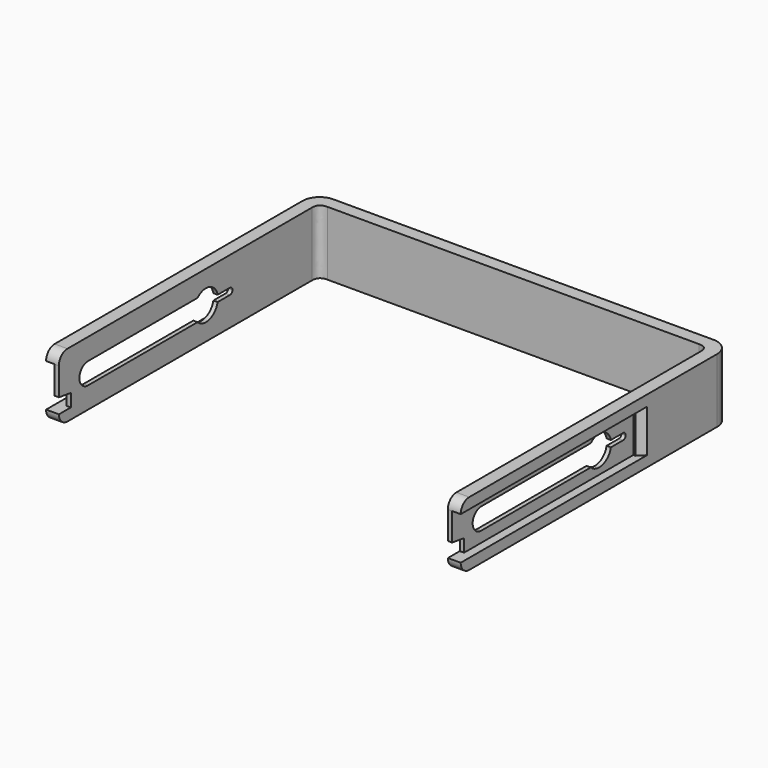
from build123d import *

# Parameters (mm, degrees)
F3_DEPTH      = 15
F4_R          = 2.5
F5_DEPTH      = 48.501
F5_DEPTH_BACK = 48.501
F6_START      = 46.5
F6_DEPTH      = 8.5
F7_START      = 2.5
F7_DEPTH      = 10
F2_W          = 73.5
F2_H          = 1
F8_DEPTH      = 0.6
F9_DEPTH      = 0.8
F10_DEPTH     = 1
F11_R         = 4
F12_T1_DEPTH  = 15


# Not quite as in the source:
# - a fillet or chamfer that OpenCascade refuses, or shapes differently, is made with other operations: its cross-section is extruded or revolved along the edge and cut away or added
# - a pattern or mirror of a feature is missing from the dataset's text; its kind, count and spacing are read off the source's solid


with BuildPart() as f3:
    # F0 (on Top) → F3 (new body)
    with BuildSketch(Plane.XY):
        Polygon((48.5, 0), (-48.5, 0), (-48.5, -79), (-45.5, -79), (-45.5, -3), (45.5, -3), (45.5, -79), (48.5, -79), (48.5, -26), (47, -26), (48.5, -24.5), align=None)
        Polygon((48.5, -26), (48.5, -24.5), (47, -26), align=None)
    extrude(amount=F3_DEPTH)

    # F4
    f4_edges = [f3.edges().sort_by_distance(p)[0] for p in [
        (-47, -79, 15),
        (-47, -79, 0),
        (47, -79, 0),
        (47, -79, 15),
    ]]
    fillet(f4_edges, radius=F4_R)

    # F1 (on Right) → F5 (cut, two sides)
    with BuildSketch(Plane.YZ) as f5_sk:
        with BuildLine():
            ThreePointArc((-38.4494897428, 5), (-39.5, 7.5), (-38.4494897428, 10))
            Line((-38.4494897428, 10), (-70.5, 10))
            ThreePointArc((-70.5, 10), (-68.732233047, 9.267766953), (-68, 7.5))
            ThreePointArc((-68, 7.5), (-68.732233047, 5.732233047), (-70.5, 5))
            Line((-70.5, 5), (-38.4494897428, 5))
        make_face()
        with BuildLine():
            ThreePointArc((-68, 7.5), (-68.732233047, 9.267766953), (-70.5, 10))
            ThreePointArc((-70.5, 10), (-73, 7.5), (-70.5, 5))
            ThreePointArc((-70.5, 5), (-68.732233047, 5.732233047), (-68, 7.5))
        make_face()
        with BuildLine():
            ThreePointArc((-32.5813014172, 6.75), (-32.5203847167, 7.1228031282), (-32.5, 7.5))
            ThreePointArc((-32.5, 7.5), (-32.5203847167, 7.8771968718), (-32.5813014172, 8.25))
            ThreePointArc((-32.5813014172, 8.25), (-34.9997668052, 10.8540324322), (-38.4494897428, 10))
            ThreePointArc((-38.4494897428, 10), (-39.5, 7.5), (-38.4494897428, 5))
            ThreePointArc((-38.4494897428, 5), (-34.9997668052, 4.1459675678), (-32.5813014172, 6.75))
        make_face()
        Polygon((-79, 6), (-79, 2.5), (-75.5, 2.5), (-75.5, 5.5), align=None)
        with BuildLine():
            ThreePointArc((-32.5813014172, 8.25), (-32.5203847167, 7.8771968718), (-32.5, 7.5))
            ThreePointArc((-32.5, 7.5), (-32.5203847167, 7.1228031282), (-32.5813014172, 6.75))
            Line((-32.5813014172, 6.75), (-29, 6.75))
            ThreePointArc((-29, 6.75), (-29.75, 7.5), (-29, 8.25))
            Line((-29, 8.25), (-32.5813014172, 8.25))
        make_face()
        with BuildLine():
            ThreePointArc((-28.25, 7.5), (-28.4696699141, 8.0303300859), (-29, 8.25))
            ThreePointArc((-29, 8.25), (-29.75, 7.5), (-29, 6.75))
            ThreePointArc((-29, 6.75), (-28.4696699141, 6.9696699141), (-28.25, 7.5))
        make_face()
    extrude(amount=-F5_DEPTH, mode=Mode.SUBTRACT)
    extrude(f5_sk.sketch, amount=F5_DEPTH_BACK, mode=Mode.SUBTRACT)

    # F1 (on Right) → F6 (cut)
    with BuildSketch(Plane.YZ.offset(F6_START)):
        Polygon((-79, 6), (-79, 2.5), (-75.5, 2.5), (-75.5, 5.5), align=None)
        Polygon((-75.5, 5.5), (-75.5, 2.5), (-26, 2.5), (-26, 12.5), (-79, 12.5), (-79, 7.5), (-79, 6), align=None)
        with BuildLine():
            ThreePointArc((-38.4494897428, 10), (-34.9997668052, 10.8540324322), (-32.5813014172, 8.25))
            Line((-32.5813014172, 8.25), (-29, 8.25))
            ThreePointArc((-29, 8.25), (-28.4696699141, 8.0303300859), (-28.25, 7.5))
            ThreePointArc((-28.25, 7.5), (-28.4696699141, 6.9696699141), (-29, 6.75))
            Line((-29, 6.75), (-32.5813014172, 6.75))
            ThreePointArc((-32.5813014172, 6.75), (-34.9997668052, 4.1459675678), (-38.4494897428, 5))
            Line((-38.4494897428, 5), (-70.5, 5))
            ThreePointArc((-70.5, 5), (-73, 7.5), (-70.5, 10))
            Line((-70.5, 10), (-38.4494897428, 10))
        make_face(mode=Mode.SUBTRACT)
        with BuildLine():
            ThreePointArc((-38.4494897428, 5), (-39.5, 7.5), (-38.4494897428, 10))
            Line((-38.4494897428, 10), (-70.5, 10))
            ThreePointArc((-70.5, 10), (-68.732233047, 9.267766953), (-68, 7.5))
            ThreePointArc((-68, 7.5), (-68.732233047, 5.732233047), (-70.5, 5))
            Line((-70.5, 5), (-38.4494897428, 5))
        make_face()
        with BuildLine():
            ThreePointArc((-68, 7.5), (-68.732233047, 9.267766953), (-70.5, 10))
            ThreePointArc((-70.5, 10), (-73, 7.5), (-70.5, 5))
            ThreePointArc((-70.5, 5), (-68.732233047, 5.732233047), (-68, 7.5))
        make_face()
        with BuildLine():
            ThreePointArc((-32.5813014172, 6.75), (-32.5203847167, 7.1228031282), (-32.5, 7.5))
            ThreePointArc((-32.5, 7.5), (-32.5203847167, 7.8771968718), (-32.5813014172, 8.25))
            ThreePointArc((-32.5813014172, 8.25), (-34.9997668052, 10.8540324322), (-38.4494897428, 10))
            ThreePointArc((-38.4494897428, 10), (-39.5, 7.5), (-38.4494897428, 5))
            ThreePointArc((-38.4494897428, 5), (-34.9997668052, 4.1459675678), (-32.5813014172, 6.75))
        make_face()
    f6 = extrude(amount=F6_DEPTH, mode=Mode.SUBTRACT)

    # F6_copies: F6 across plane
    add(f6.mirror(Plane(origin=(0, 0, 0), x_dir=(0, 0, -1), z_dir=(-1, 0, 0))), mode=Mode.SUBTRACT)

    # F0 (on Top) → F7 (cut)
    with BuildSketch(Plane.XY.offset(F7_START)):
        Polygon((48.5, -26), (48.5, -24.5), (47, -26), align=None)
    f7 = extrude(amount=F7_DEPTH, mode=Mode.SUBTRACT)

    # F7_copies: F7 across plane
    add(f7.mirror(Plane(origin=(0, 0, 0), x_dir=(0, 0, -1), z_dir=(-1, 0, 0))), mode=Mode.SUBTRACT)

    # F2 (on Front) → F8 (join)
    with BuildSketch(Plane.XZ):
        with Locations((0, 12.5)):
            Rectangle(F2_W, F2_H)
        with Locations((-0.0531907369, 2.5001414637)):
            Rectangle(F2_W, F2_H)
    extrude(amount=-F8_DEPTH)

    # F2 (on Front) → F9 (join)
    with BuildSketch(Plane.XZ):
        with Locations((-0.0106381474, 10.5000282927)):
            Rectangle(F2_W, F2_H)
        with Locations((-0.0425525895, 4.500113171)):
            Rectangle(F2_W, F2_H)
    extrude(amount=-F9_DEPTH)

    # F2 (on Front) → F10 (join)
    with BuildSketch(Plane.XZ):
        with Locations((-0.0212762948, 8.5000565855)):
            Rectangle(F2_W, F2_H)
        with Locations((-0.0319144421, 6.5000848782)):
            Rectangle(F2_W, F2_H)
    extrude(amount=-F10_DEPTH)

    # F11
    f11_edges = [f3.edges().sort_by_distance(p)[0] for p in [
        (48.5, 0, 7.5),
        (-48.5, 0, 7.5),
    ]]
    fillet(f11_edges, radius=F11_R)

    # F12: fillet of radius 2 on 2 edges, made by hand

    # F12_s2 → F12_t1 (join)
    with BuildSketch(Plane.XY):
        with BuildLine():
            add(Edge.make_bspline(
                [(-45.5, -5), (-45.5, -3), (-43.5, -3)],
                knots=[0, 0, 0, 1, 1, 1], degree=2, weights=[1, 1, 1]))
            Line((-43.5, -3), (-45.5, -3))
            Line((-45.5, -3), (-45.5, -5))
        make_face()
        with BuildLine():
            add(Edge.make_bspline(
                [(43.5, -3), (45.5, -3), (45.5, -5)],
                knots=[0, 0, 0, 1, 1, 1], degree=2, weights=[1, 1, 1]))
            Line((45.5, -5), (45.5, -3))
            Line((45.5, -3), (43.5, -3))
        make_face()
    extrude(amount=F12_T1_DEPTH)


solid = f3.part
